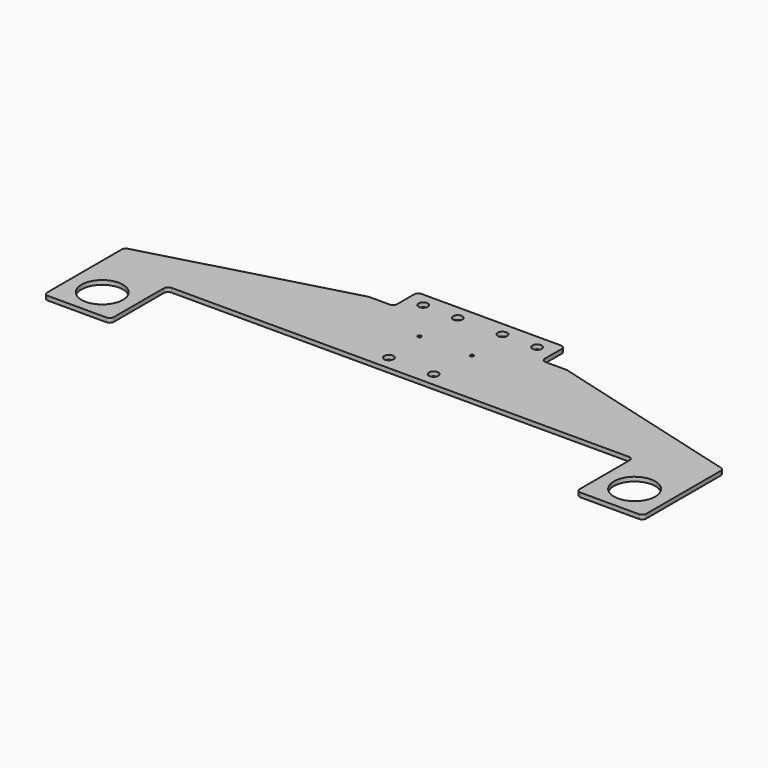
from build123d import *

# Parameters (mm, degrees)
F0_W     = 79
F0_H     = 84
F0_W_2   = 175
F0_H_2   = 35
F1_DEPTH = 5
F2_R     = 5
F3_R     = 5
F6_D     = 4.1
F8_D     = 49
F9_D     = 11


# Not quite as in the source:
# - a feature names something its author has since deleted; it is built from what else it names


with BuildPart() as f1:
    # F0 (on Top) → F1 (new body)
    with BuildSketch(Plane.XY):
        Polygon((-87.5, 50), (-117.5, 50), (-355, -15), (-355, -50), (-276, -50), (276, -50), (355, -50), (355, -15), (117.5, 50), (87.5, 50), align=None)
        with Locations((-315.5, -92)):
            Rectangle(F0_W, F0_H)
        with Locations((315.5, -92)):
            Rectangle(F0_W, F0_H)
        with Locations((0, 67.5)):
            Rectangle(F0_W_2, F0_H_2)
    extrude(amount=F1_DEPTH)

    # F2
    f2_edges = [f1.edges().sort_by_distance(p)[0] for p in [
        (-355, -134, 2.5),
        (-276, -134, 2.5),
        (276, -134, 2.5),
        (355, -134, 2.5),
        (355, -15, 2.5),
        (-355, -15, 2.5),
        (-276, -50, 2.5),
        (276, -50, 2.5),
        (-87.5, 50, 2.5),
        (-87.5, 85, 2.5),
        (87.5, 85, 2.5),
        (87.5, 50, 2.5),
    ]]
    fillet(f2_edges, radius=F2_R)

    # F3
    f3_edges = [f1.edges().sort_by_distance(p)[0] for p in [
        (117.5, 50, 2.5),
        (-117.5, 50, 2.5),
    ]]
    fillet(f3_edges, radius=F3_R)

    # F6 (through all)
    with Locations(Plane(origin=(0, 0, 0), x_dir=(1, 0, 0), z_dir=(0, 0, -1))):
        with Locations((-31, -17.5), (31, -17.5)):
            Hole(F6_D / 2)

    # F8 (through all)
    with Locations(Plane(origin=(0, 0, 0), x_dir=(1, 0, 0), z_dir=(0, 0, -1))):
        with Locations((-315.5, 97), (315.5, 97)):
            Hole(F8_D / 2)

    # F9 (through all)
    with Locations(Plane(origin=(0, 0, 0), x_dir=(1, 0, 0), z_dir=(0, 0, -1))):
        with Locations((-67.5, -68.5), (67.5, -68.5), (-26.5, -68.5), (26.5, -68.5), (-26.5, 33.5), (26.5, 33.5)):
            Hole(F9_D / 2)


solid = f1.part
